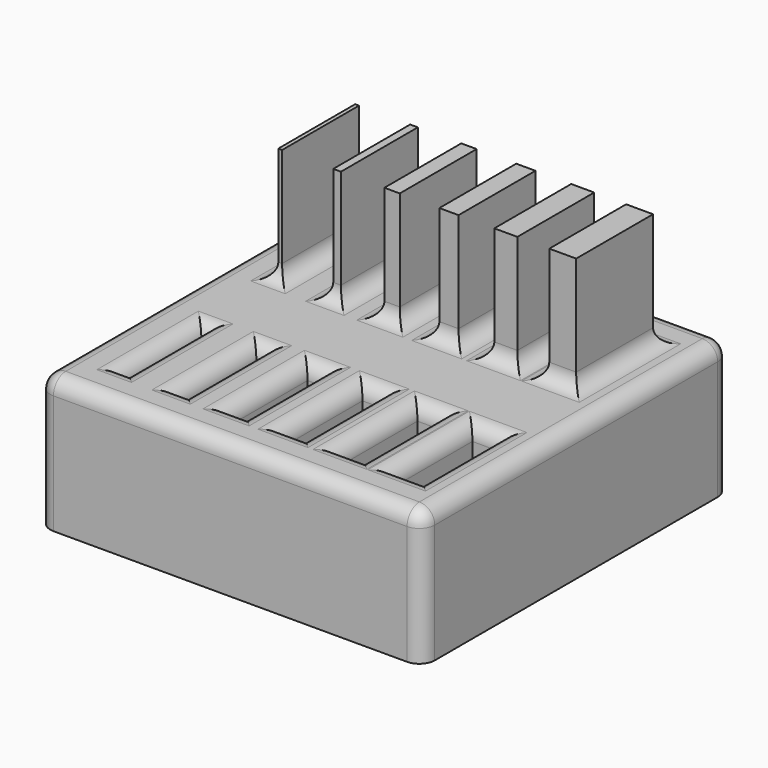
from build123d import *

# Parameters (mm, degrees)
F0_W      = 20
F0_H      = 20
F1_DEPTH  = 3
F2_W      = 0.2
F2_H      = 5
F3_DEPTH  = 10
F4_DEPTH  = 0.1
F5_DEPTH  = 0.4
F6_DEPTH  = 0.5
F7_DEPTH  = 0.6
F8_DEPTH  = 0.7
F9_DEPTH  = 4
F10_W     = 0.2
F10_H     = 5
F10_W_2   = 0.4
F10_W_3   = 0.8
F10_W_4   = 1
F10_W_5   = 1.2
F10_W_6   = 1.4
F11_DEPTH = 7
F12_R     = 0.8


with BuildPart() as f1:
    # F0 (on Top) → F1 (new body)
    with BuildSketch(Plane.XY):
        Rectangle(F0_W, F0_H)
    extrude(amount=F1_DEPTH)

    # F2 (on face) → F3 (join)
    with BuildSketch(Plane.XY.offset(3)):
        with Locations((-7.4, 5)):
            Rectangle(F2_W, F2_H)
        with Locations((-4.44, 5)):
            Rectangle(F2_W, F2_H)
        with Locations((-1.48, 5)):
            Rectangle(F2_W, F2_H)
        with Locations((1.48, 5)):
            Rectangle(F2_W, F2_H)
        with Locations((4.44, 5)):
            Rectangle(F2_W, F2_H)
        with Locations((7.4, 5)):
            Rectangle(F2_W, F2_H)
    extrude(amount=F3_DEPTH)

    # F4 (add, symmetric): faces of the model
    f4_faces = [f1.faces().sort_by_distance(p)[0] for p in [
        (-4.54, 5, 8),
        (-4.34, 5, 8),
    ]]
    extrude(f4_faces, amount=F4_DEPTH, both=True, dir=(-1, 0, 0))

    # F5 (add, symmetric): a face of the model
    f5_faces = [f1.faces().sort_by_distance(p)[0] for p in [
        (-1.58, 5, 8),
    ]]
    extrude(f5_faces, amount=F5_DEPTH, both=True)

    # F6 (add, symmetric): a face of the model
    f6_faces = [f1.faces().sort_by_distance(p)[0] for p in [
        (1.38, 5, 8),
    ]]
    extrude(f6_faces, amount=F6_DEPTH, both=True)

    # F7 (add, symmetric): a face of the model
    f7_faces = [f1.faces().sort_by_distance(p)[0] for p in [
        (4.34, 5, 8),
    ]]
    extrude(f7_faces, amount=F7_DEPTH, both=True)

    # F8 (add, symmetric): a face of the model
    f8_faces = [f1.faces().sort_by_distance(p)[0] for p in [
        (7.3, 5, 8),
    ]]
    extrude(f8_faces, amount=F8_DEPTH, both=True)

    # F9 (add): a face of the model
    f9_faces = [f1.faces().sort_by_distance(p)[0] for p in [
        (-0.16384, -0.3333333333, 3),
    ]]
    extrude(f9_faces, amount=F9_DEPTH)

    # F10 (on face) → F11 (cut, through all)
    with BuildSketch(Plane.XY.offset(7)):
        with Locations((-7.4, -5)):
            Rectangle(F10_W, F10_H)
        with Locations((-4.44, -5)):
            Rectangle(F10_W_2, F10_H)
        with Locations((-1.58, -5)):
            Rectangle(F10_W_3, F10_H)
        with Locations((1.38, -5)):
            Rectangle(F10_W_4, F10_H)
        with Locations((4.34, -5)):
            Rectangle(F10_W_5, F10_H)
        with Locations((7.3, -5)):
            Rectangle(F10_W_6, F10_H)
    extrude(amount=-F11_DEPTH, mode=Mode.SUBTRACT)

    # F12
    f12_edges = [f1.edges().sort_by_distance(p)[0] for p in [
        (10, -10, 3.5),
        (-10, -10, 3.5),
        (-10, 10, 3.5),
        (10, 10, 3.5),
        (-10, 0, 7),
        (0, 10, 7),
        (0, -10, 7),
        (10, 0, 7),
        (-7.5, 5, 7),
        (-7.3, 5, 7),
        (-4.64, 5, 7),
        (-4.24, 5, 7),
        (-1.98, 5, 7),
        (-1.18, 5, 7),
        (0.88, 5, 7),
        (1.88, 5, 7),
        (3.74, 5, 7),
        (6.6, 5, 7),
        (4.94, 5, 7),
        (8, 5, 7),
        (-7.4, 7.5, 7),
        (-7.4, 2.5, 7),
        (-4.44, 2.5, 7),
        (-1.58, 2.5, 7),
        (1.38, 2.5, 7),
        (4.34, 2.5, 7),
        (7.3, 2.5, 7),
        (7.3, -2.5, 7),
        (8, -5, 7),
        (6.6, -5, 7),
        (7.3, -7.5, 7),
        (4.94, -5, 7),
        (4.34, -2.5, 7),
        (4.34, -7.5, 7),
        (3.74, -5, 7),
        (1.88, -5, 7),
        (1.38, -2.5, 7),
        (1.38, -7.5, 7),
        (0.88, -5, 7),
        (-1.18, -5, 7),
        (-1.98, -5, 7),
        (-1.58, -2.5, 7),
        (-1.58, -7.5, 7),
        (-4.24, -5, 7),
        (-4.44, -2.5, 7),
        (-4.64, -5, 7),
        (-4.44, -7.5, 7),
        (-7.3, -5, 7),
        (-7.5, -5, 7),
        (-7.4, -2.5, 7),
        (-7.4, -7.5, 7),
        (-4.44, 7.5, 7),
        (-1.58, 7.5, 7),
        (1.38, 7.5, 7),
        (4.34, 7.5, 7),
        (7.3, 7.5, 7),
    ]]
    fillet(f12_edges, radius=F12_R)


solid = f1.part
